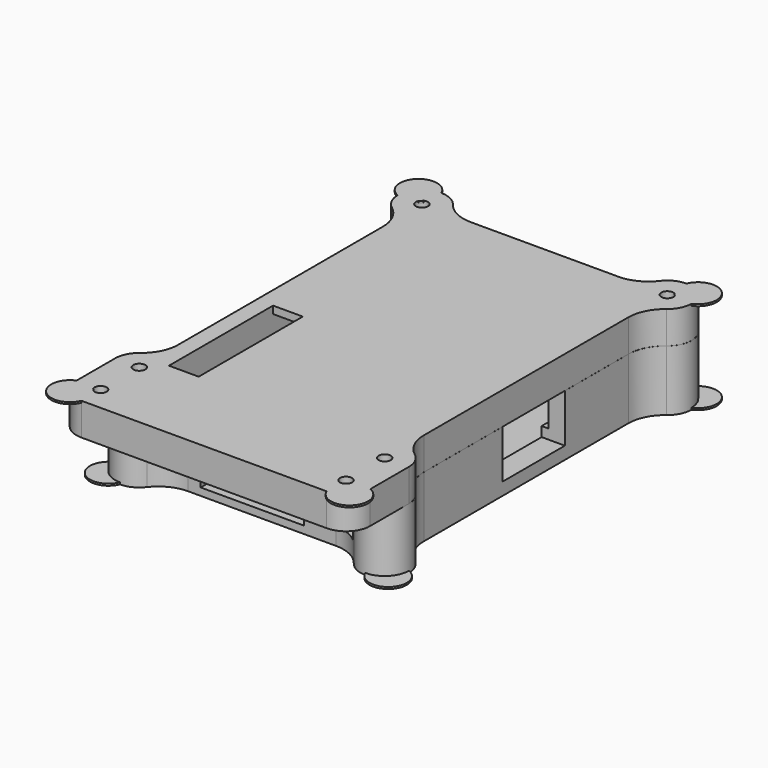
from build123d import *

# Parameters (mm, degrees)
F0_W           = 66
F0_H           = 95
F1_DEPTH       = 23.1
F2_W           = 56
F2_H           = 85
F3_DEPTH       = 17.1
F4_W           = 53.5
F4_H           = 85
F5_DEPTH       = 4
F6_W           = 27.8
F6_H           = 4
F6_W_2         = 11.5
F6_H_2         = 8.5
F7_DEPTH       = 5
F8_W           = 16.4
F8_H           = 14
F8_W_2         = 14.25
F8_H_2         = 16.5
F9_DEPTH       = 5
F10_W          = 21
F10_H          = 13
F11_DEPTH      = 6.25
F12_R          = 4.35
F12_R_2        = 5.15
F13_DEPTH      = 5
F14_W          = 57.15
F14_H          = 86.15
F15_DEPTH      = 17.1
F16_W          = 53.5
F16_H          = 0.575
F17_DEPTH      = 4
F18_W          = 66
F18_H          = 95
F19_DEPTH      = 2
F20_R          = 6.5
F21_DEPTH      = 25.1
F22_R          = 1.625
F23_DEPTH      = 25.101
F24_T1_DEPTH   = 25.1
F24_T3_DEPTH   = 4
F24_T5_DEPTH   = 7.1
F24_T10_DEPTH  = 25.1
F24_T16_DEPTH  = 25.1
F24_T22_DEPTH  = 25.1
F24_T29_DEPTH  = 25.1
F24_T35_DEPTH  = 25.1
F24_T41_DEPTH  = 20.561011871
F24_T46_DEPTH  = 23.661011871
F25_W          = 120
F25_H          = 0.01
F26_DEPTH      = 72.501
F26_DEPTH_BACK = 6.501
F27_W          = 8
F27_H          = 35
F28_DEPTH      = 8.726
F29_R          = 2.5
F30_DEPTH      = 14.365
F31_R          = 1.625
F32_DEPTH      = 2
F33_W          = 5.55
F33_H          = 3
F34_DEPTH      = 6.725
F35_R          = 2.5
F36_DEPTH      = 16.365
F37_R          = 5
F38_DEPTH      = 0.5
F39_R          = 1.625
F40_DEPTH      = 8.725
F41_R          = 5
F42_DEPTH      = 0.5


# Not quite as in the source:
# - a fillet or chamfer that OpenCascade refuses, or shapes differently, is made with other operations: its cross-section is extruded or revolved along the edge and cut away or added


with BuildPart() as f1:
    # F0 (on Top) → F1 (new body)
    with BuildSketch(Plane.XY):
        Rectangle(F0_W, F0_H)
    extrude(amount=F1_DEPTH)

    # F2 (on face) → F3 (cut)
    with BuildSketch(Plane.XY.offset(23.1)):
        Rectangle(F2_W, F2_H)
    extrude(amount=-F3_DEPTH, mode=Mode.SUBTRACT)

    # F4 (on face) → F5 (cut)
    with BuildSketch(Plane.XY.offset(6)):
        Rectangle(F4_W, F4_H)
    extrude(amount=-F5_DEPTH, mode=Mode.SUBTRACT)

    # F6 (on face) → F7 (cut, through all)
    with BuildSketch(Plane.XZ.offset(47.5)):
        with Locations((-2.6, 4)):
            Rectangle(F6_W, F6_H)
        with Locations((20.6, 8.8)):
            Rectangle(F6_W_2, F6_H_2)
    extrude(amount=-F7_DEPTH, mode=Mode.SUBTRACT)

    # F8 (on face) → F9 (cut, through all)
    with BuildSketch(Plane(origin=(0, 47.5, 0), x_dir=(-1, 0, 0), z_dir=(0, 1, 0))):
        with Locations((-18.3, 14.1)):
            Rectangle(F8_W, F8_H)
        with Locations((2.575, 15.35)):
            Rectangle(F8_W_2, F8_H_2)
    extrude(amount=-F9_DEPTH, mode=Mode.SUBTRACT)

    # F10 (on face) → F11 (cut, through all)
    with BuildSketch(Plane.YZ.offset(33)):
        with Locations((2.55, 9.875)):
            Rectangle(F10_W, F10_H)
    extrude(amount=-F11_DEPTH, mode=Mode.SUBTRACT)

    # F12 (on face) → F13 (cut, through all)
    with BuildSketch(Plane(origin=(-33, 0, 0), x_dir=(0, -1, 0), z_dir=(-1, 0, 0))):
        with Locations((-22, 13.95)):
            Circle(F12_R)
        with Locations((-3.25, 15.75)):
            Circle(F12_R_2)
    extrude(amount=-F13_DEPTH, mode=Mode.SUBTRACT)

    # F14 (on face) → F15 (cut, through all)
    with BuildSketch(Plane.XY.offset(23.1)):
        Rectangle(F14_W, F14_H)
    extrude(amount=-F15_DEPTH, mode=Mode.SUBTRACT)

    # F16 (on face) → F17 (cut, through all)
    with BuildSketch(Plane.XY.offset(6)):
        with Locations((0, 42.7875)):
            Rectangle(F16_W, F16_H)
        with Locations((0, -42.7875)):
            Rectangle(F16_W, F16_H)
    extrude(amount=-F17_DEPTH, mode=Mode.SUBTRACT)

    # F18 (on face) → F19 (join)
    with BuildSketch(Plane.XY.offset(23.1)):
        Rectangle(F18_W, F18_H)
    extrude(amount=F19_DEPTH)

    # F20 (on face) → F21 (join, through all)
    with BuildSketch(Plane.XY.offset(25.1)):
        with Locations((-33, 47.5)):
            Circle(F20_R)
        with Locations((33, 47.5)):
            Circle(F20_R)
        with Locations((33, -47.5)):
            Circle(F20_R)
        with Locations((-33, -47.5)):
            Circle(F20_R)
    extrude(amount=-F21_DEPTH)

    # F22 (on face) → F23 (cut, through all)
    with BuildSketch(Plane.XY.offset(25.1)):
        with Locations((-33, -47.5)):
            Circle(F22_R)
        with Locations((33, -47.5)):
            Circle(F22_R)
        with Locations((33, 47.5)):
            Circle(F22_R)
        with Locations((-33, 47.5)):
            Circle(F22_R)
    extrude(amount=-F23_DEPTH, mode=Mode.SUBTRACT)

    # F24: fillet of radius 10 on 9 edges, made by hand

    # F24_s2 → F24_t1 (join)
    with BuildSketch(Plane.XY):
        with BuildLine():
            ThreePointArc((-33, 34.3755952516), (-34.0388041924, 38.8137220746), (-36.9393939394, 42.3297799476))
            ThreePointArc((-36.9393939394, 42.3297799476), (-35.078890288, 41.341411268), (-33, 41))
            Line((-33, 41), (-33, 34.3755952516))
        make_face()
        with BuildLine():
            ThreePointArc((-36.9393939394, -42.3297799476), (-34.0388041924, -38.8137220746), (-33, -34.3755952516))
            Line((-33, -34.3755952516), (-33, -41))
            ThreePointArc((-33, -41), (-35.078890288, -41.341411268), (-36.9393939394, -42.3297799476))
        make_face()
        with BuildLine():
            ThreePointArc((-19.8755952516, -47.5), (-24.3137220746, -48.5388041924), (-27.8297799476, -51.4393939394))
            ThreePointArc((-27.8297799476, -51.4393939394), (-26.841411268, -49.578890288), (-26.5, -47.5))
            Line((-26.5, -47.5), (-19.8755952516, -47.5))
        make_face()
        with BuildLine():
            ThreePointArc((36.9393939394, -42.3297799476), (34.0388041924, -38.8137220746), (33, -34.3755952516))
            Line((33, -34.3755952516), (33, -41))
            ThreePointArc((33, -41), (35.078890288, -41.341411268), (36.9393939394, -42.3297799476))
        make_face()
        with BuildLine():
            ThreePointArc((33, 34.3755952516), (34.0388041924, 38.8137220746), (36.9393939394, 42.3297799476))
            ThreePointArc((36.9393939394, 42.3297799476), (35.078890288, 41.341411268), (33, 41))
            Line((33, 41), (33, 34.3755952516))
        make_face()
        with BuildLine():
            ThreePointArc((-19.8755952516, 47.5), (-24.3137220746, 48.5388041924), (-27.8297799476, 51.4393939394))
            ThreePointArc((-27.8297799476, 51.4393939394), (-26.841411268, 49.578890288), (-26.5, 47.5))
            Line((-26.5, 47.5), (-19.8755952516, 47.5))
        make_face()
    extrude(amount=F24_T1_DEPTH)

    # F24_s4 → F24_t3 (join)
    with BuildSketch(Plane.XY.offset(21.1)):
        with BuildLine():
            ThreePointArc((27.8297799476, 51.4393939394), (24.3137220746, 48.5388041924), (19.8755952516, 47.5))
            Line((19.8755952516, 47.5), (26.5, 47.5))
            ThreePointArc((26.5, 47.5), (26.841411268, 49.578890288), (27.8297799476, 51.4393939394))
        make_face()
    extrude(amount=F24_T3_DEPTH)

    # F24_s6 → F24_t5 (join)
    with BuildSketch(Plane.XY):
        with BuildLine():
            ThreePointArc((27.8297799476, 51.4393939394), (24.3137220746, 48.5388041924), (19.8755952516, 47.5))
            Line((19.8755952516, 47.5), (26.5, 47.5))
            ThreePointArc((26.5, 47.5), (26.841411268, 49.578890288), (27.8297799476, 51.4393939394))
        make_face()
    extrude(amount=F24_T5_DEPTH)


with BuildPart() as f24_tool8:
    # F24_s9 → F24_t10 (new body)
    with BuildSketch(Plane.XY):
        with BuildLine():
            ThreePointArc((27.8297799476, -51.4393939394), (24.3137220746, -48.5388041924), (19.8755952516, -47.5))
            Line((19.8755952516, -47.5), (26.5, -47.5))
            ThreePointArc((26.5, -47.5), (26.841411268, -49.578890288), (27.8297799476, -51.4393939394))
        make_face()
    extrude(amount=F24_T10_DEPTH)

    split(bisect_by=Plane.XY.offset(4.55), keep=Keep.BOTTOM)

    split(bisect_by=Plane.YZ.offset(26.35), keep=Keep.TOP)


with BuildPart() as f1_1:
    add(f1.part)

    # F24_t7: union F24_tool8
    add(f24_tool8.part)


with BuildPart() as f24_tool14:
    # F24_s15 → F24_t16 (new body)
    with BuildSketch(Plane.XY):
        with BuildLine():
            ThreePointArc((27.8297799476, -51.4393939394), (24.3137220746, -48.5388041924), (19.8755952516, -47.5))
            Line((19.8755952516, -47.5), (26.5, -47.5))
            ThreePointArc((26.5, -47.5), (26.841411268, -49.578890288), (27.8297799476, -51.4393939394))
        make_face()
    extrude(amount=F24_T16_DEPTH)

    split(bisect_by=Plane.XY.offset(4.55), keep=Keep.BOTTOM)

    split(bisect_by=Plane.YZ.offset(26.35), keep=Keep.BOTTOM)


with BuildPart() as f1_2:
    add(f1_1.part)

    # F24_t13: union F24_tool14
    add(f24_tool14.part)


with BuildPart() as f24_tool20:
    # F24_s21 → F24_t22 (new body)
    with BuildSketch(Plane.XY):
        with BuildLine():
            ThreePointArc((27.8297799476, -51.4393939394), (24.3137220746, -48.5388041924), (19.8755952516, -47.5))
            Line((19.8755952516, -47.5), (26.5, -47.5))
            ThreePointArc((26.5, -47.5), (26.841411268, -49.578890288), (27.8297799476, -51.4393939394))
        make_face()
    extrude(amount=F24_T22_DEPTH)

    split(bisect_by=Plane.XY.offset(4.55), keep=Keep.TOP)

    split(bisect_by=Plane.YZ.offset(26.35), keep=Keep.TOP)

    split(bisect_by=Plane.XY.offset(13.05), keep=Keep.BOTTOM)


with BuildPart() as f1_3:
    add(f1_2.part)

    # F24_t19: union F24_tool20
    add(f24_tool20.part)


with BuildPart() as f24_tool27:
    # F24_s28 → F24_t29 (new body)
    with BuildSketch(Plane.XY):
        with BuildLine():
            ThreePointArc((27.8297799476, -51.4393939394), (24.3137220746, -48.5388041924), (19.8755952516, -47.5))
            Line((19.8755952516, -47.5), (26.5, -47.5))
            ThreePointArc((26.5, -47.5), (26.841411268, -49.578890288), (27.8297799476, -51.4393939394))
        make_face()
    extrude(amount=F24_T29_DEPTH)

    split(bisect_by=Plane.YZ.offset(26.35), keep=Keep.TOP)

    split(bisect_by=Plane.XY.offset(13.05), keep=Keep.TOP)


with BuildPart() as f1_4:
    add(f1_3.part)

    # F24_t26: union F24_tool27
    add(f24_tool27.part)


with BuildPart() as f24_tool33:
    # F24_s34 → F24_t35 (new body)
    with BuildSketch(Plane.XY):
        with BuildLine():
            ThreePointArc((27.8297799476, -51.4393939394), (24.3137220746, -48.5388041924), (19.8755952516, -47.5))
            Line((19.8755952516, -47.5), (26.5, -47.5))
            ThreePointArc((26.5, -47.5), (26.841411268, -49.578890288), (27.8297799476, -51.4393939394))
        make_face()
    extrude(amount=F24_T35_DEPTH)

    split(bisect_by=Plane.YZ.offset(26.35), keep=Keep.BOTTOM)

    split(bisect_by=Plane.XY.offset(13.05), keep=Keep.TOP)


with BuildPart() as f1_5:
    add(f1_4.part)

    # F24_t32: union F24_tool33
    add(f24_tool33.part)


with BuildPart() as f24_tool39:
    # F24_s40 → F24_t41 (new body)
    with BuildSketch(Plane.XY.offset(4.538988129)):
        with BuildLine():
            ThreePointArc((27.8297799476, 51.4393939394), (24.3137220746, 48.5388041924), (19.8755952516, 47.5))
            Line((19.8755952516, 47.5), (26.5, 47.5))
            ThreePointArc((26.5, 47.5), (26.841411268, 49.578890288), (27.8297799476, 51.4393939394))
        make_face()
    extrude(amount=F24_T41_DEPTH)

    split(bisect_by=Plane.XY.offset(7.1), keep=Keep.BOTTOM)


with BuildPart() as f1_6:
    add(f1_5.part)

    # F24_t38: union F24_tool39
    add(f24_tool39.part)


with BuildPart() as f24_tool44:
    # F24_s45 → F24_t46 (new body)
    with BuildSketch(Plane.XY):
        with BuildLine():
            ThreePointArc((27.8297799476, 51.4393939394), (24.3137220746, 48.5388041924), (19.8755952516, 47.5))
            Line((19.8755952516, 47.5), (26.5, 47.5))
            ThreePointArc((26.5, 47.5), (26.841411268, 49.578890288), (27.8297799476, 51.4393939394))
        make_face()
    extrude(amount=F24_T46_DEPTH)

    split(bisect_by=Plane.XY.offset(21.1), keep=Keep.TOP)


with BuildPart() as f1_7:
    add(f1_6.part)

    # F24_t43: union F24_tool44
    add(f24_tool44.part)

    # F25 (on face) → F26 (cut, two sides)
    with BuildSketch(Plane.YZ.offset(33)) as f26_sk:
        with Locations((-1.7188391089, 16.37)):
            Rectangle(F25_W, F25_H)
    extrude(amount=-F26_DEPTH, mode=Mode.SUBTRACT)
    extrude(f26_sk.sketch, amount=F26_DEPTH_BACK, mode=Mode.SUBTRACT)

    # F27 (on face) → F28 (cut, through all)
    with BuildSketch(Plane.XY.offset(25.1)):
        with Locations((-24.575, -25.575)):
            Rectangle(F27_W, F27_H)
    extrude(amount=-F28_DEPTH, mode=Mode.SUBTRACT)

    # F29 (on face) → F30 (cut, through all)
    with BuildSketch(Plane.XY.offset(16.365)):
        with Locations((-33, 47.5)):
            Circle(F29_R)
        with Locations((33, 47.5)):
            Circle(F29_R)
        with Locations((-33, -47.5)):
            Circle(F29_R)
        with Locations((33, -47.5)):
            Circle(F29_R)
    extrude(amount=-F30_DEPTH, mode=Mode.SUBTRACT)

    # F31 (on face) → F32 (join, through all)
    with BuildSketch(Plane(origin=(0, 0, 0), x_dir=(1, 0, 0), z_dir=(0, 0, -1))):
        with Locations((-33, -47.5)):
            Circle(F31_R)
        with Locations((-33, 47.5)):
            Circle(F31_R)
        with Locations((33, 47.5)):
            Circle(F31_R)
        with Locations((33, -47.5)):
            Circle(F31_R)
    extrude(amount=-F32_DEPTH)

    # F33 (on face) → F34 (join, through all)
    with BuildSketch(Plane(origin=(0, 0, 16.375), x_dir=(1, 0, 0), z_dir=(0, 0, -1))):
        with Locations((7.325, -41.575)):
            Rectangle(F33_W, F33_H)
    extrude(amount=-F34_DEPTH)

    # F35 (on face) → F36 (cut, through all)
    with BuildSketch(Plane(origin=(0, 0, 0), x_dir=(1, 0, 0), z_dir=(0, 0, -1))):
        with Locations((33, 47.5)):
            Circle(F35_R)
        with Locations((-33, 47.5)):
            Circle(F35_R)
        with Locations((33, -47.5)):
            Circle(F35_R)
        with Locations((-33, -47.5)):
            Circle(F35_R)
    extrude(amount=-F36_DEPTH, mode=Mode.SUBTRACT)

    # F37 (on face) → F38 (join)
    with BuildSketch(Plane(origin=(0, 0, 0), x_dir=(1, 0, 0), z_dir=(0, 0, -1))):
        with Locations((37.5961940777, 52.0961940777)):
            Circle(F37_R)
        with Locations((37.5961940777, -52.0961940777)):
            Circle(F37_R)
        with Locations((-37.5961940777, -52.0961940777)):
            Circle(F37_R)
        with Locations((-37.5961940777, 52.0961940777)):
            Circle(F37_R)
    extrude(amount=-F38_DEPTH)

    # F39 (on face) → F40 (join, through all)
    with BuildSketch(Plane.XY.offset(25.1)):
        with BuildLine():
            ThreePointArc((-27.8297799476, -51.4393939394), (-35.078890288, -53.658588732), (-39.5, -47.5))
            Line((-39.5, -47.5), (-39.5, -60.5))
            ThreePointArc((-39.5, -60.5), (-37.5961940777, -65.0961940777), (-33, -67))
            Line((-33, -67), (33, -67))
            ThreePointArc((33, -67), (37.5961940777, -65.0961940777), (39.5, -60.5))
            Line((39.5, -60.5), (39.5, -47.5))
            ThreePointArc((39.5, -47.5), (35.078890288, -53.658588732), (27.8297799476, -51.4393939394))
            ThreePointArc((27.8297799476, -51.4393939394), (24.3137220746, -48.5388041924), (19.8755952516, -47.5))
            Line((19.8755952516, -47.5), (-19.8755952516, -47.5))
            ThreePointArc((-19.8755952516, -47.5), (-24.3137220746, -48.5388041924), (-27.8297799476, -51.4393939394))
        make_face()
        with Locations((-33, -60.5)):
            Circle(F39_R, mode=Mode.SUBTRACT)
        with Locations((33, -60.5)):
            Circle(F39_R, mode=Mode.SUBTRACT)
    extrude(amount=-F40_DEPTH)

    # F41 (on face) → F42 (join)
    with BuildSketch(Plane.XY.offset(25.1)):
        with Locations((-37.5961940777, -65.0961940777)):
            Circle(F41_R)
        with Locations((-37.5961940777, 52.0961940777)):
            Circle(F41_R)
        with Locations((37.5961940777, 52.0961940777)):
            Circle(F41_R)
        with Locations((37.5961940777, -65.0961940777)):
            Circle(F41_R)
    extrude(amount=-F42_DEPTH)


solid = f1_7.part
